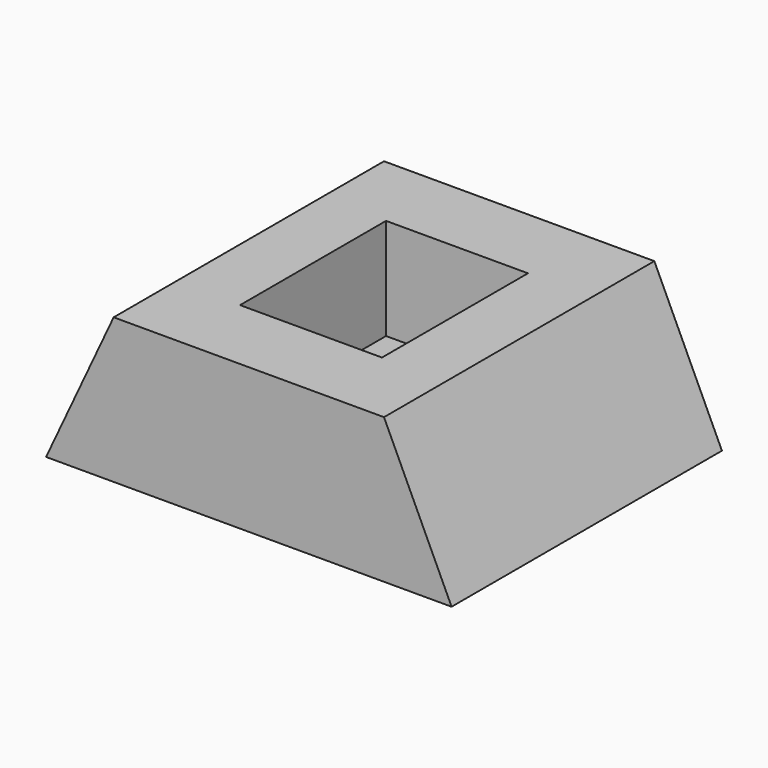
from build123d import *

# Parameters (mm, degrees)
F1_DEPTH = 250
F2_W     = 105
F2_H     = 135
F3_DEPTH = 75


# Not quite as in the source:
# - a feature names something its author has since deleted; it is built from what else it names


with BuildPart() as f1:
    # F0 (on Front) → F1 (new body)
    with BuildSketch(Plane.XZ):
        Polygon((-74.1169694188, 46.7042212901), (-124.1169694188, -60.5211247353), (175.8830305812, -60.5211247353), (125.8830305812, 46.7042212901), align=None)
    extrude(amount=F1_DEPTH)

    # F2 (on face) → F3 (cut)
    with BuildSketch(Plane.XY.offset(46.7042212901)):
        with Locations((25.8830305812, -125)):
            Rectangle(F2_W, F2_H)
    extrude(amount=-F3_DEPTH, mode=Mode.SUBTRACT)


solid = f1.part
